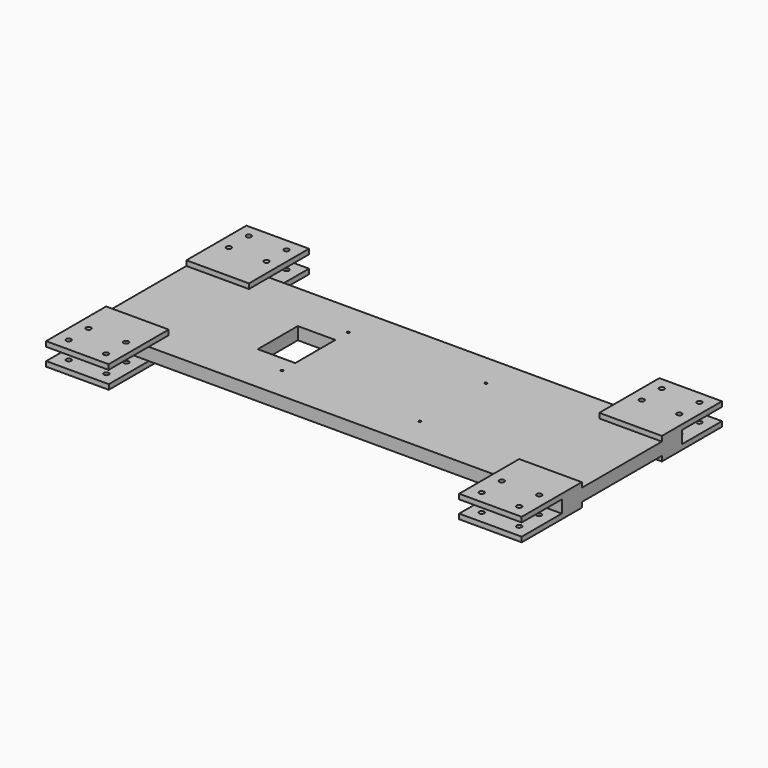
from build123d import *

# Parameters (mm, degrees)
F0_W     = 190
F0_H     = 60
F1_DEPTH = 5
F2_W     = 25
F2_H     = 20
F2_H_2   = 10
F2_W_2   = 24.9426496029
F3_DEPTH = 2
F4_W     = 25
F4_H     = 20
F4_H_2   = 10
F5_DEPTH = 2


with BuildPart() as f1:
    # F0 (on Top) → F1 (new body)
    with BuildSketch(Plane.XY):
        Rectangle(F0_W, F0_H)
        with BuildLine():
            Line((27, -16.5), (-27, -16.5))
            ThreePointArc((-27, -16.5), (-27.8535533906, -16.8535533906), (-27.5, -16))
            Line((-27.5, -16), (-27.5, -10))
            Line((-27.5, -10), (-42.4774698913, -10))
            Line((-42.4774698913, -10), (-42.4774698913, 10))
            Line((-42.4774698913, 10), (-27.5, 10))
            Line((-27.5, 10), (-27.5, 16))
            ThreePointArc((-27.5, 16), (-27.8535533906, 16.8535533906), (-27, 16.5))
            Line((-27, 16.5), (27, 16.5))
            ThreePointArc((27, 16.5), (27.5, 17), (28, 16.5))
            ThreePointArc((28, 16.5), (27.8535533906, 16.1464466094), (27.5, 16))
            Line((27.5, 16), (27.5, -16))
            ThreePointArc((27.5, -16), (27.8535533906, -16.1464466094), (28, -16.5))
            ThreePointArc((28, -16.5), (27.5, -17), (27, -16.5))
        make_face(mode=Mode.SUBTRACT)
        with BuildLine():
            ThreePointArc((-27.5, -16), (-27.1464466094, -16.1464466094), (-27, -16.5))
            Line((-27, -16.5), (27, -16.5))
            ThreePointArc((27, -16.5), (27.1464466094, -16.1464466094), (27.5, -16))
            Line((27.5, -16), (27.5, 16))
            ThreePointArc((27.5, 16), (27.1464466094, 16.1464466094), (27, 16.5))
            Line((27, 16.5), (-27, 16.5))
            ThreePointArc((-27, 16.5), (-27.1464466094, 16.1464466094), (-27.5, 16))
            Line((-27.5, 16), (-27.5, 10))
            Line((-27.5, 10), (-27.4774698913, 10))
            Line((-27.4774698913, 10), (-27.4774698913, -10))
            Line((-27.4774698913, -10), (-27.5, -10))
            Line((-27.5, -10), (-27.5, -16))
        make_face()
    extrude(amount=F1_DEPTH)

    # F2 (on face) → F3 (join)
    with BuildSketch(Plane.XY.offset(5)):
        Polygon((-95, -30), (-95, -20), (-95.0573503971, -20), (-95.0573503971, -50), (-70.0573503971, -50), (-70.0573503971, -30), align=None)
        with BuildLine():
            Line((-76.0573503971, -45), (-89.0573503971, -45))
            ThreePointArc((-89.0573503971, -45), (-90.7644571783, -45.7071067812), (-90.0573503971, -44))
            Line((-90.0573503971, -44), (-90.0573503971, -36))
            ThreePointArc((-90.0573503971, -36), (-90.7644571783, -34.2928932188), (-89.0573503971, -35))
            Line((-89.0573503971, -35), (-76.0573503971, -35))
            ThreePointArc((-76.0573503971, -35), (-75.0573503971, -34), (-74.0573503971, -35))
            ThreePointArc((-74.0573503971, -35), (-74.3502436159, -35.7071067812), (-75.0573503971, -36))
            Line((-75.0573503971, -36), (-75.0573503971, -44))
            ThreePointArc((-75.0573503971, -44), (-74.3502436159, -44.2928932188), (-74.0573503971, -45))
            ThreePointArc((-74.0573503971, -45), (-75.0573503971, -46), (-76.0573503971, -45))
        make_face(mode=Mode.SUBTRACT)
        with Locations((-82.5, 40)):
            Rectangle(F2_W, F2_H)
        with BuildLine():
            ThreePointArc((-90, 44), (-90.7071067812, 45.7071067812), (-89, 45))
            Line((-89, 45), (-76, 45))
            ThreePointArc((-76, 45), (-75, 46), (-74, 45))
            ThreePointArc((-74, 45), (-74.2928932188, 44.2928932188), (-75, 44))
            Line((-75, 44), (-75, 36))
            ThreePointArc((-75, 36), (-74.2928932188, 35.7071067812), (-74, 35))
            ThreePointArc((-74, 35), (-75, 34), (-76, 35))
            Line((-76, 35), (-89, 35))
            ThreePointArc((-89, 35), (-90.7071067812, 34.2928932188), (-90, 36))
            Line((-90, 36), (-90, 44))
        make_face(mode=Mode.SUBTRACT)
        with Locations((82.5, 40)):
            Rectangle(F2_W, F2_H)
        with BuildLine():
            ThreePointArc((75, 44), (74.2928932188, 45.7071067812), (76, 45))
            Line((76, 45), (89, 45))
            ThreePointArc((89, 45), (90, 46), (91, 45))
            ThreePointArc((91, 45), (90.7071067812, 44.2928932188), (90, 44))
            Line((90, 44), (90, 36))
            ThreePointArc((90, 36), (90.7071067812, 35.7071067812), (91, 35))
            ThreePointArc((91, 35), (90, 34), (89, 35))
            Line((89, 35), (76, 35))
            ThreePointArc((76, 35), (74.2928932188, 34.2928932188), (75, 36))
            Line((75, 36), (75, 44))
        make_face(mode=Mode.SUBTRACT)
        with Locations((82.5, -40)):
            Rectangle(F2_W, F2_H)
        with BuildLine():
            Line((89, -45), (76, -45))
            ThreePointArc((76, -45), (74.2928932188, -45.7071067812), (75, -44))
            Line((75, -44), (75, -36))
            ThreePointArc((75, -36), (74.2928932188, -34.2928932188), (76, -35))
            Line((76, -35), (89, -35))
            ThreePointArc((89, -35), (90, -34), (91, -35))
            ThreePointArc((91, -35), (90.7071067812, -35.7071067812), (90, -36))
            Line((90, -36), (90, -44))
            ThreePointArc((90, -44), (90.7071067812, -44.2928932188), (91, -45))
            ThreePointArc((91, -45), (90, -46), (89, -45))
        make_face(mode=Mode.SUBTRACT)
        with Locations((-82.5, 25)):
            Rectangle(F2_W, F2_H_2)
        with Locations((82.5, 25)):
            Rectangle(F2_W, F2_H_2)
        with Locations((82.5, -25)):
            Rectangle(F2_W, F2_H_2)
        with Locations((-82.5286751986, -25)):
            Rectangle(F2_W_2, F2_H_2)
        with BuildLine():
            Line((-76, 45), (-89, 45))
            ThreePointArc((-89, 45), (-89.2928932188, 44.2928932188), (-90, 44))
            Line((-90, 44), (-90, 36))
            ThreePointArc((-90, 36), (-89.2928932188, 35.7071067812), (-89, 35))
            Line((-89, 35), (-76, 35))
            ThreePointArc((-76, 35), (-75.7071067812, 35.7071067812), (-75, 36))
            Line((-75, 36), (-75, 44))
            ThreePointArc((-75, 44), (-75.7071067812, 44.2928932188), (-76, 45))
        make_face()
        with BuildLine():
            Line((89, 45), (76, 45))
            ThreePointArc((76, 45), (75.7071067812, 44.2928932188), (75, 44))
            Line((75, 44), (75, 36))
            ThreePointArc((75, 36), (75.7071067812, 35.7071067812), (76, 35))
            Line((76, 35), (89, 35))
            ThreePointArc((89, 35), (89.2928932188, 35.7071067812), (90, 36))
            Line((90, 36), (90, 44))
            ThreePointArc((90, 44), (89.2928932188, 44.2928932188), (89, 45))
        make_face()
        with BuildLine():
            ThreePointArc((75, -44), (75.7071067812, -44.2928932188), (76, -45))
            Line((76, -45), (89, -45))
            ThreePointArc((89, -45), (89.2928932188, -44.2928932188), (90, -44))
            Line((90, -44), (90, -36))
            ThreePointArc((90, -36), (89.2928932188, -35.7071067812), (89, -35))
            Line((89, -35), (76, -35))
            ThreePointArc((76, -35), (75.7071067812, -35.7071067812), (75, -36))
            Line((75, -36), (75, -44))
        make_face()
        with BuildLine():
            ThreePointArc((-90.0573503971, -44), (-89.3502436159, -44.2928932188), (-89.0573503971, -45))
            Line((-89.0573503971, -45), (-76.0573503971, -45))
            ThreePointArc((-76.0573503971, -45), (-75.7644571783, -44.2928932188), (-75.0573503971, -44))
            Line((-75.0573503971, -44), (-75.0573503971, -36))
            ThreePointArc((-75.0573503971, -36), (-75.7644571783, -35.7071067812), (-76.0573503971, -35))
            Line((-76.0573503971, -35), (-89.0573503971, -35))
            ThreePointArc((-89.0573503971, -35), (-89.3502436159, -35.7071067812), (-90.0573503971, -36))
            Line((-90.0573503971, -36), (-90.0573503971, -44))
        make_face()
    extrude(amount=F3_DEPTH)

    # F4 (on face) → F5 (join)
    with BuildSketch(Plane(origin=(0, 0, 0), x_dir=(1, 0, 0), z_dir=(0, 0, -1))):
        with Locations((-82.5, 40)):
            Rectangle(F4_W, F4_H)
        with BuildLine():
            ThreePointArc((-90, 44), (-90.7071067812, 45.7071067812), (-89, 45))
            Line((-89, 45), (-76, 45))
            ThreePointArc((-76, 45), (-75, 46), (-74, 45))
            ThreePointArc((-74, 45), (-74.2928932188, 44.2928932188), (-75, 44))
            Line((-75, 44), (-75, 36))
            ThreePointArc((-75, 36), (-74.2928932188, 35.7071067812), (-74, 35))
            ThreePointArc((-74, 35), (-75, 34), (-76, 35))
            Line((-76, 35), (-89, 35))
            ThreePointArc((-89, 35), (-90.7071067812, 34.2928932188), (-90, 36))
            Line((-90, 36), (-90, 44))
        make_face(mode=Mode.SUBTRACT)
        with Locations((82.5, 40)):
            Rectangle(F4_W, F4_H)
        with BuildLine():
            ThreePointArc((75, 44), (74.2928932188, 45.7071067812), (76, 45))
            Line((76, 45), (89, 45))
            ThreePointArc((89, 45), (90, 46), (91, 45))
            ThreePointArc((91, 45), (90.7071067812, 44.2928932188), (90, 44))
            Line((90, 44), (90, 36))
            ThreePointArc((90, 36), (90.7071067812, 35.7071067812), (91, 35))
            ThreePointArc((91, 35), (90, 34), (89, 35))
            Line((89, 35), (76, 35))
            ThreePointArc((76, 35), (74.2928932188, 34.2928932188), (75, 36))
            Line((75, 36), (75, 44))
        make_face(mode=Mode.SUBTRACT)
        with Locations((82.5, -40)):
            Rectangle(F4_W, F4_H)
        with BuildLine():
            Line((89, -45), (76, -45))
            ThreePointArc((76, -45), (74.2928932188, -45.7071067812), (75, -44))
            Line((75, -44), (75, -36.0721963992))
            ThreePointArc((75, -36.0721963992), (74.2928932188, -34.365089618), (76, -35.0721963992))
            Line((76, -35.0721963992), (89, -35.0721963992))
            ThreePointArc((89, -35.0721963992), (90, -34.0721963992), (91, -35.0721963992))
            ThreePointArc((91, -35.0721963992), (90.7071067812, -35.7793031804), (90, -36.0721963992))
            Line((90, -36.0721963992), (90, -44))
            ThreePointArc((90, -44), (90.7071067812, -44.2928932188), (91, -45))
            ThreePointArc((91, -45), (90, -46), (89, -45))
        make_face(mode=Mode.SUBTRACT)
        with Locations((-82.5, -40)):
            Rectangle(F4_W, F4_H)
        with BuildLine():
            Line((-76, -45), (-89, -45))
            ThreePointArc((-89, -45), (-90.7071067812, -45.7071067812), (-90, -44))
            Line((-90, -44), (-90, -36))
            ThreePointArc((-90, -36), (-90.7071067812, -34.2928932188), (-89, -35))
            Line((-89, -35), (-76, -35))
            ThreePointArc((-76, -35), (-75, -34), (-74, -35))
            ThreePointArc((-74, -35), (-74.2928932188, -35.7071067812), (-75, -36))
            Line((-75, -36), (-75, -44))
            ThreePointArc((-75, -44), (-74.2928932188, -44.2928932188), (-74, -45))
            ThreePointArc((-74, -45), (-75, -46), (-76, -45))
        make_face(mode=Mode.SUBTRACT)
        with Locations((-82.5, 25)):
            Rectangle(F4_W, F4_H_2)
        with Locations((82.5, 25)):
            Rectangle(F4_W, F4_H_2)
        with Locations((82.5, -25)):
            Rectangle(F4_W, F4_H_2)
        with Locations((-82.5, -25)):
            Rectangle(F4_W, F4_H_2)
        with BuildLine():
            Line((-76, 45), (-89, 45))
            ThreePointArc((-89, 45), (-89.2928932188, 44.2928932188), (-90, 44))
            Line((-90, 44), (-90, 36))
            ThreePointArc((-90, 36), (-89.2928932188, 35.7071067812), (-89, 35))
            Line((-89, 35), (-76, 35))
            ThreePointArc((-76, 35), (-75.7071067812, 35.7071067812), (-75, 36))
            Line((-75, 36), (-75, 44))
            ThreePointArc((-75, 44), (-75.7071067812, 44.2928932188), (-76, 45))
        make_face()
        with BuildLine():
            Line((89, 45), (76, 45))
            ThreePointArc((76, 45), (75.7071067812, 44.2928932188), (75, 44))
            Line((75, 44), (75, 36))
            ThreePointArc((75, 36), (75.7071067812, 35.7071067812), (76, 35))
            Line((76, 35), (89, 35))
            ThreePointArc((89, 35), (89.2928932188, 35.7071067812), (90, 36))
            Line((90, 36), (90, 44))
            ThreePointArc((90, 44), (89.2928932188, 44.2928932188), (89, 45))
        make_face()
        with BuildLine():
            ThreePointArc((-90, -44), (-89.2928932188, -44.2928932188), (-89, -45))
            Line((-89, -45), (-76, -45))
            ThreePointArc((-76, -45), (-75.7071067812, -44.2928932188), (-75, -44))
            Line((-75, -44), (-75, -36))
            ThreePointArc((-75, -36), (-75.7071067812, -35.7071067812), (-76, -35))
            Line((-76, -35), (-89, -35))
            ThreePointArc((-89, -35), (-89.2928932188, -35.7071067812), (-90, -36))
            Line((-90, -36), (-90, -44))
        make_face()
        with BuildLine():
            ThreePointArc((75, -44), (75.7071067812, -44.2928932188), (76, -45))
            Line((76, -45), (89, -45))
            ThreePointArc((89, -45), (89.2928932188, -44.2928932188), (90, -44))
            Line((90, -44), (90, -36.0721963992))
            ThreePointArc((90, -36.0721963992), (89.2928932188, -35.7793031804), (89, -35.0721963992))
            Line((89, -35.0721963992), (76, -35.0721963992))
            ThreePointArc((76, -35.0721963992), (75.7071067812, -35.7793031804), (75, -36.0721963992))
            Line((75, -36.0721963992), (75, -44))
        make_face()
    extrude(amount=F5_DEPTH)


solid = f1.part
